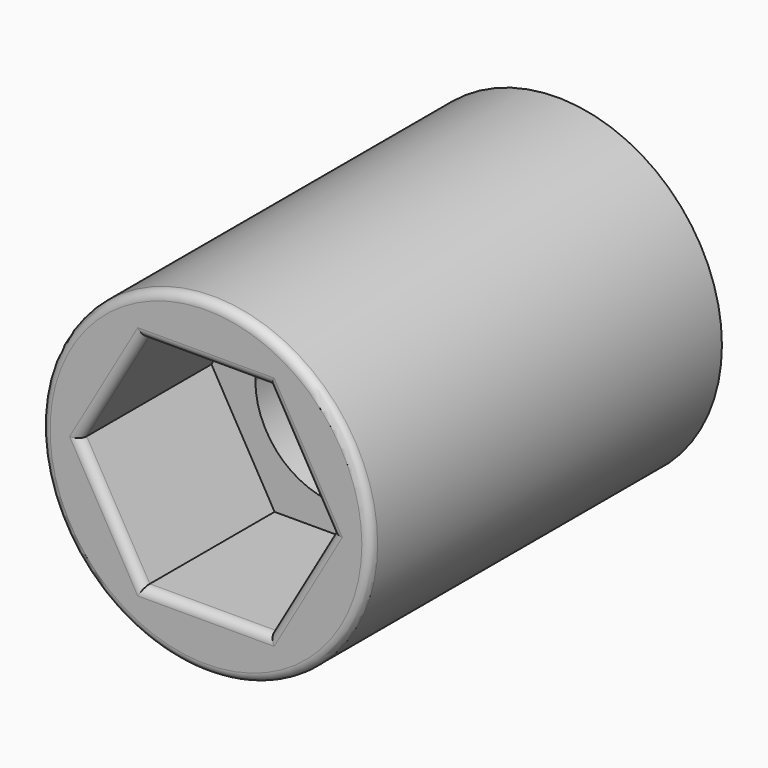
from build123d import *

# Parameters (mm, degrees)
F0_R      = 9.525
F1_DEPTH  = 25.4
F3_DEPTH  = 50
F5_DEPTH  = 25.401
F6_DEPTH  = 9.398
F7_DEPTH  = 12.7
F8_DEPTH  = 11.0998
F10_DEPTH = 9.525
F11_R     = 0.508


# Not quite as in the source:
# - an extrude ends at something that could not be found from the text; its depth is read off the source's solid


with BuildPart() as f1:
    # F0 (on Front) → F1 (new body)
    with BuildSketch(Plane.XZ):
        Circle(F0_R)
    extrude(amount=F1_DEPTH)

    # F2 (on Front) → F3 (cut, through all)
    with BuildSketch(Plane.XZ):
        with BuildLine():
            ThreePointArc((4.7625, 0), (3.3675960454, 3.3675960454), (0, 4.7625))
            ThreePointArc((0, 4.7625), (-3.3675960454, 3.3675960454), (-4.7625, 0))
            ThreePointArc((-4.7625, 0), (-3.3675960454, -3.3675960454), (0, -4.7625))
            ThreePointArc((0, -4.7625), (3.3675960454, -3.3675960454), (4.7625, 0))
        make_face()
    extrude(amount=-F3_DEPTH, mode=Mode.SUBTRACT)

    # F4 (on face) → F5 (cut, through all)
    with BuildSketch(Plane(origin=(0, 0, 0), x_dir=(-1, 0, 0), z_dir=(0, 1, 0))):
        with BuildLine():
            ThreePointArc((-4.7625, 0), (-3.3675960454, -3.3675960454), (0, -4.7625))
            ThreePointArc((0, -4.7625), (3.3675960454, -3.3675960454), (4.7625, 0))
            ThreePointArc((4.7625, 0), (3.3675960454, 3.3675960454), (0, 4.7625))
            ThreePointArc((0, 4.7625), (-3.3675960454, 3.3675960454), (-4.7625, 0))
        make_face()
    extrude(amount=-F5_DEPTH, mode=Mode.SUBTRACT)

    # F2 (on Front) → F6 (cut)
    with BuildSketch(Plane.XZ):
        with BuildLine():
            Line((4.7625, 0), (4.7625, 4.7625))
            Line((4.7625, 4.7625), (0, 4.7625))
            ThreePointArc((0, 4.7625), (3.3675960454, 3.3675960454), (4.7625, 0))
        make_face()
        with BuildLine():
            ThreePointArc((-4.7625, 0), (-3.3675960454, 3.3675960454), (0, 4.7625))
            Line((0, 4.7625), (-4.7625, 4.7625))
            Line((-4.7625, 4.7625), (-4.7625, 0))
        make_face()
        with BuildLine():
            ThreePointArc((4.7625, 0), (3.3675960454, 3.3675960454), (0, 4.7625))
            ThreePointArc((0, 4.7625), (-3.3675960454, 3.3675960454), (-4.7625, 0))
            ThreePointArc((-4.7625, 0), (-3.3675960454, -3.3675960454), (0, -4.7625))
            ThreePointArc((0, -4.7625), (3.3675960454, -3.3675960454), (4.7625, 0))
        make_face()
        with BuildLine():
            Line((4.7625, -4.7625), (4.7625, 0))
            ThreePointArc((4.7625, 0), (3.3675960454, -3.3675960454), (0, -4.7625))
            Line((0, -4.7625), (4.7625, -4.7625))
        make_face()
        with BuildLine():
            ThreePointArc((0, -4.7625), (-3.3675960454, -3.3675960454), (-4.7625, 0))
            Line((-4.7625, 0), (-4.7625, -4.7625))
            Line((-4.7625, -4.7625), (0, -4.7625))
        make_face()
    extrude(amount=-F6_DEPTH, mode=Mode.SUBTRACT)

    # F2 (on Front) → F7 (cut)
    with BuildSketch(Plane.XZ):
        with BuildLine():
            Line((4.7625, 0), (4.7625, 4.7625))
            Line((4.7625, 4.7625), (0, 4.7625))
            ThreePointArc((0, 4.7625), (3.3675960454, 3.3675960454), (4.7625, 0))
        make_face()
        with BuildLine():
            ThreePointArc((-4.7625, 0), (-3.3675960454, 3.3675960454), (0, 4.7625))
            Line((0, 4.7625), (-4.7625, 4.7625))
            Line((-4.7625, 4.7625), (-4.7625, 0))
        make_face()
        with BuildLine():
            ThreePointArc((4.7625, 0), (3.3675960454, 3.3675960454), (0, 4.7625))
            ThreePointArc((0, 4.7625), (-3.3675960454, 3.3675960454), (-4.7625, 0))
            ThreePointArc((-4.7625, 0), (-3.3675960454, -3.3675960454), (0, -4.7625))
            ThreePointArc((0, -4.7625), (3.3675960454, -3.3675960454), (4.7625, 0))
        make_face()
        with BuildLine():
            Line((4.7625, -4.7625), (4.7625, 0))
            ThreePointArc((4.7625, 0), (3.3675960454, -3.3675960454), (0, -4.7625))
            Line((0, -4.7625), (4.7625, -4.7625))
        make_face()
        with BuildLine():
            ThreePointArc((0, -4.7625), (-3.3675960454, -3.3675960454), (-4.7625, 0))
            Line((-4.7625, 0), (-4.7625, -4.7625))
            Line((-4.7625, -4.7625), (0, -4.7625))
        make_face()
    extrude(amount=-F7_DEPTH, mode=Mode.SUBTRACT)

    # F2 (on Front) → F8 (cut)
    with BuildSketch(Plane.XZ):
        with BuildLine():
            Line((4.7625, 0), (4.7625, 4.7625))
            Line((4.7625, 4.7625), (0, 4.7625))
            ThreePointArc((0, 4.7625), (3.3675960454, 3.3675960454), (4.7625, 0))
        make_face()
        with BuildLine():
            ThreePointArc((-4.7625, 0), (-3.3675960454, 3.3675960454), (0, 4.7625))
            Line((0, 4.7625), (-4.7625, 4.7625))
            Line((-4.7625, 4.7625), (-4.7625, 0))
        make_face()
        with BuildLine():
            ThreePointArc((4.7625, 0), (3.3675960454, 3.3675960454), (0, 4.7625))
            ThreePointArc((0, 4.7625), (-3.3675960454, 3.3675960454), (-4.7625, 0))
            ThreePointArc((-4.7625, 0), (-3.3675960454, -3.3675960454), (0, -4.7625))
            ThreePointArc((0, -4.7625), (3.3675960454, -3.3675960454), (4.7625, 0))
        make_face()
        with BuildLine():
            Line((4.7625, -4.7625), (4.7625, 0))
            ThreePointArc((4.7625, 0), (3.3675960454, -3.3675960454), (0, -4.7625))
            Line((0, -4.7625), (4.7625, -4.7625))
        make_face()
        with BuildLine():
            ThreePointArc((0, -4.7625), (-3.3675960454, -3.3675960454), (-4.7625, 0))
            Line((-4.7625, 0), (-4.7625, -4.7625))
            Line((-4.7625, -4.7625), (0, -4.7625))
        make_face()
    extrude(amount=F8_DEPTH, mode=Mode.SUBTRACT)

    # F9 (on face) → F10 (cut)
    with BuildSketch(Plane.XZ.offset(25.4)):
        Polygon((3.65125, 6.3241505111), (-3.65125, 6.3241505111), (-7.3025, 0), (-3.65125, -6.3241505111), (3.65125, -6.3241505111), (7.3025, 0), align=None)
    extrude(amount=-F10_DEPTH, mode=Mode.SUBTRACT)

    # F11
    f11_edges = [f1.edges().sort_by_distance(p)[0] for p in [
        (-9.525, -25.4, 0),
        (-5.476875, -25.4, 3.162075),
        (0, -25.4, 6.324151),
        (5.476875, -25.4, 3.162075),
        (-5.476875, -25.4, -3.162075),
        (0, -25.4, -6.324151),
        (5.476875, -25.4, -3.162075),
    ]]
    fillet(f11_edges, radius=F11_R)


solid = f1.part
